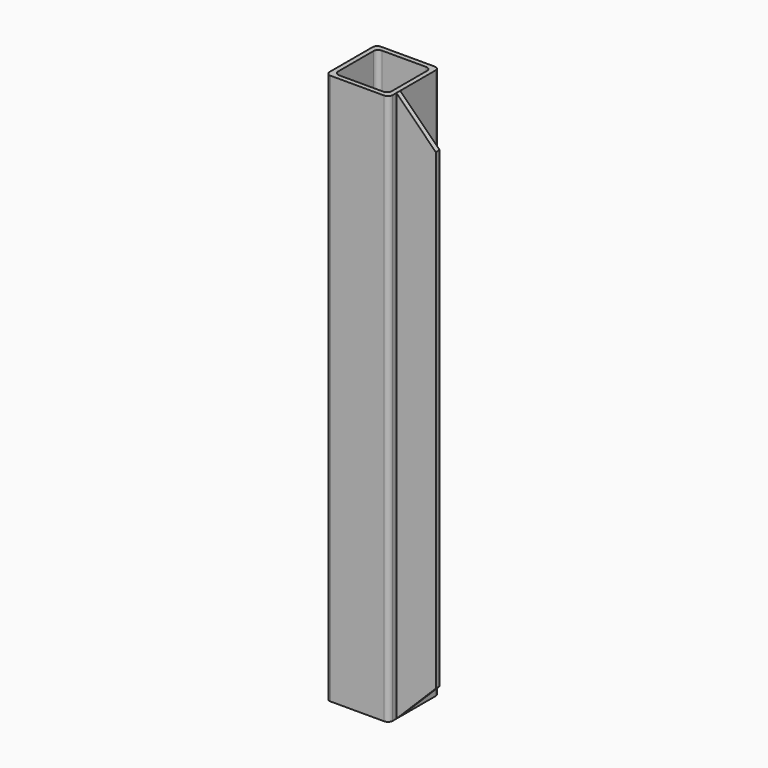
from build123d import *

# Parameters (mm, degrees)
F1_DEPTH = 175
F2_W     = 3
F2_H     = 350
F3_DEPTH = 25
F5_DEPTH = 34.001


# Not quite as in the source:
# - a pattern or mirror of a feature is missing from the dataset's text; its kind, count and spacing are read off the source's solid


with BuildPart() as f1:
    # F0 (on Top) → F1 (new body, symmetric)
    with BuildSketch(Plane.XY):
        with BuildLine():
            ThreePointArc((20, 17), (19.1213203436, 19.1213203436), (17, 20))
            Line((17, 20), (-17, 20))
            ThreePointArc((-17, 20), (-19.1213203436, 19.1213203436), (-20, 17))
            Line((-20, 17), (-20, -17))
            ThreePointArc((-20, -17), (-19.1213203436, -19.1213203436), (-17, -20))
            Line((-17, -20), (17, -20))
            ThreePointArc((17, -20), (19.1213203436, -19.1213203436), (20, -17))
            Line((20, -17), (20, 17))
        make_face()
        with BuildLine():
            ThreePointArc((14, 17), (16.1213203436, 16.1213203436), (17, 14))
            Line((17, 14), (17, -14))
            ThreePointArc((17, -14), (16.1213203436, -16.1213203436), (14, -17))
            Line((14, -17), (-14, -17))
            ThreePointArc((-14, -17), (-16.1213203436, -16.1213203436), (-17, -14))
            Line((-17, -14), (-17, 14))
            ThreePointArc((-17, 14), (-16.1213203436, 16.1213203436), (-14, 17))
            Line((-14, 17), (14, 17))
        make_face(mode=Mode.SUBTRACT)
    extrude(amount=F1_DEPTH, both=True)

    # F2 (on face) → F3 (join)
    with BuildSketch(Plane.YZ.offset(20)):
        with Locations((-12.5, 0)):
            Rectangle(F2_W, F2_H)
    extrude(amount=F3_DEPTH)

    # F4 (on face) → F5 (cut, through all)
    with BuildSketch(Plane.XZ.offset(14)):
        Polygon((45, 175), (20, 175), (45, 150), align=None)
    f5 = extrude(amount=-F5_DEPTH, mode=Mode.SUBTRACT)

    # F5_copies: F5 across plane
    add(f5.mirror(Plane(origin=(0, 0, 0), x_dir=(-1, 0, 0), z_dir=(0, 0, -1))), mode=Mode.SUBTRACT)


solid = f1.part
